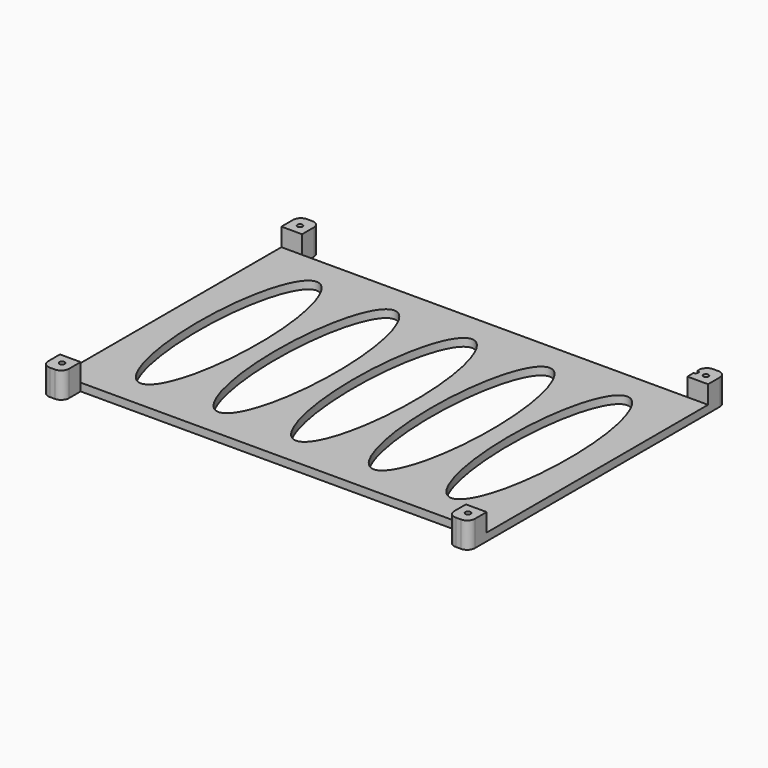
from build123d import *

# Parameters (mm, degrees)
F0_W     = 4
F0_H     = 106.96
F0_H_2   = 4
F0_W_2   = 148.9
F1_DEPTH = 3
F2_DEPTH = 10
F3_D     = 2
F5_DEPTH = 25


# Not quite as in the source:
# - a feature names something its author has since deleted; it is built from what else it names


with BuildPart() as f1:
    # F0 (on Top) → F1 (new body)
    with BuildSketch(Plane.XY):
        with Locations((-80.45, 0)):
            Rectangle(F0_W, F0_H)
        with Locations((-76.45, 55.48)):
            Rectangle(F0_W, F0_H_2)
        Rectangle(F0_W_2, F0_H)
        with Locations((-76.45, 0)):
            Rectangle(F0_W, F0_H)
        with BuildLine():
            ThreePointArc((82.45, 59.135), (81.5713203436, 61.2563203436), (79.45, 62.135))
            Line((79.45, 62.135), (77.45, 62.135))
            ThreePointArc((77.45, 62.135), (75.3286796564, 61.2563203436), (74.45, 59.135))
            Line((74.45, 59.135), (74.45, 57.48))
            Line((74.45, 57.48), (78.45, 57.48))
            Line((78.45, 57.48), (78.45, 53.48))
            Line((78.45, 53.48), (82.45, 53.48))
            Line((82.45, 53.48), (82.45, 59.135))
        make_face()
        with Locations((76.45, 55.48)):
            Rectangle(F0_W, F0_H_2)
        with Locations((76.45, 0)):
            Rectangle(F0_W, F0_H)
        with Locations((80.45, 0)):
            Rectangle(F0_W, F0_H)
        with Locations((76.45, -55.48)):
            Rectangle(F0_W, F0_H_2)
        with BuildLine():
            Line((82.45, -59.135), (82.45, -53.48))
            Line((82.45, -53.48), (78.45, -53.48))
            Line((78.45, -53.48), (78.45, -57.48))
            Line((78.45, -57.48), (74.45, -57.48))
            Line((74.45, -57.48), (74.45, -59.135))
            ThreePointArc((74.45, -59.135), (75.3286796564, -61.2563203436), (77.45, -62.135))
            Line((77.45, -62.135), (79.45, -62.135))
            ThreePointArc((79.45, -62.135), (81.5713203436, -61.2563203436), (82.45, -59.135))
        make_face()
        with BuildLine():
            Line((-78.45, -57.48), (-78.45, -53.48))
            Line((-78.45, -53.48), (-82.45, -53.48))
            Line((-82.45, -53.48), (-82.45, -59.135))
            ThreePointArc((-82.45, -59.135), (-81.5713203436, -61.2563203436), (-79.45, -62.135))
            Line((-79.45, -62.135), (-77.45, -62.135))
            ThreePointArc((-77.45, -62.135), (-75.3286796564, -61.2563203436), (-74.45, -59.135))
            Line((-74.45, -59.135), (-74.45, -57.48))
            Line((-74.45, -57.48), (-78.45, -57.48))
        make_face()
        with Locations((-76.45, -55.48)):
            Rectangle(F0_W, F0_H_2)
        with BuildLine():
            Line((-82.45, 53.48), (-78.45, 53.48))
            Line((-78.45, 53.48), (-78.45, 57.48))
            Line((-78.45, 57.48), (-74.45, 57.48))
            Line((-74.45, 57.48), (-74.45, 59.135))
            ThreePointArc((-74.45, 59.135), (-75.3286796564, 61.2563203436), (-77.45, 62.135))
            Line((-77.45, 62.135), (-79.45, 62.135))
            ThreePointArc((-79.45, 62.135), (-81.5713203436, 61.2563203436), (-82.45, 59.135))
            Line((-82.45, 59.135), (-82.45, 53.48))
        make_face()
    extrude(amount=F1_DEPTH)

    # F0 (on Top) → F2 (join)
    with BuildSketch(Plane.XY):
        with BuildLine():
            ThreePointArc((82.45, 59.135), (81.5713203436, 61.2563203436), (79.45, 62.135))
            Line((79.45, 62.135), (77.45, 62.135))
            ThreePointArc((77.45, 62.135), (75.3286796564, 61.2563203436), (74.45, 59.135))
            Line((74.45, 59.135), (74.45, 57.48))
            Line((74.45, 57.48), (78.45, 57.48))
            Line((78.45, 57.48), (78.45, 53.48))
            Line((78.45, 53.48), (82.45, 53.48))
            Line((82.45, 53.48), (82.45, 59.135))
        make_face()
        with Locations((76.45, 55.48)):
            Rectangle(F0_W, F0_H_2)
        with BuildLine():
            Line((-82.45, 53.48), (-78.45, 53.48))
            Line((-78.45, 53.48), (-78.45, 57.48))
            Line((-78.45, 57.48), (-74.45, 57.48))
            Line((-74.45, 57.48), (-74.45, 59.135))
            ThreePointArc((-74.45, 59.135), (-75.3286796564, 61.2563203436), (-77.45, 62.135))
            Line((-77.45, 62.135), (-79.45, 62.135))
            ThreePointArc((-79.45, 62.135), (-81.5713203436, 61.2563203436), (-82.45, 59.135))
            Line((-82.45, 59.135), (-82.45, 53.48))
        make_face()
        with Locations((-76.45, 55.48)):
            Rectangle(F0_W, F0_H_2)
        with BuildLine():
            Line((82.45, -59.135), (82.45, -53.48))
            Line((82.45, -53.48), (78.45, -53.48))
            Line((78.45, -53.48), (78.45, -57.48))
            Line((78.45, -57.48), (74.45, -57.48))
            Line((74.45, -57.48), (74.45, -59.135))
            ThreePointArc((74.45, -59.135), (75.3286796564, -61.2563203436), (77.45, -62.135))
            Line((77.45, -62.135), (79.45, -62.135))
            ThreePointArc((79.45, -62.135), (81.5713203436, -61.2563203436), (82.45, -59.135))
        make_face()
        with Locations((76.45, -55.48)):
            Rectangle(F0_W, F0_H_2)
        with BuildLine():
            Line((-78.45, -57.48), (-78.45, -53.48))
            Line((-78.45, -53.48), (-82.45, -53.48))
            Line((-82.45, -53.48), (-82.45, -59.135))
            ThreePointArc((-82.45, -59.135), (-81.5713203436, -61.2563203436), (-79.45, -62.135))
            Line((-79.45, -62.135), (-77.45, -62.135))
            ThreePointArc((-77.45, -62.135), (-75.3286796564, -61.2563203436), (-74.45, -59.135))
            Line((-74.45, -59.135), (-74.45, -57.48))
            Line((-74.45, -57.48), (-78.45, -57.48))
        make_face()
        with Locations((-76.45, -55.48)):
            Rectangle(F0_W, F0_H_2)
    extrude(amount=F2_DEPTH)

    # F3 (through all)
    with Locations(Plane(origin=(0, 0, 0), x_dir=(1, 0, 0), z_dir=(0, 0, -1))):
        with Locations((74.45, -57.48), (78.45, -57.48), (78.45, 57.48), (-78.45, 57.48), (-78.45, -57.48)):
            Hole(F3_D / 2)

    # F4 (on face) → F5 (cut)
    with BuildSketch(Plane.XY.offset(3)):
        with BuildLine():
            add(Edge.make_bspline(
                [(-60, 42.5), (-80.0186509611, 42.5), (-70.0093254806, -21.25), (-60, -85), (-49.9906745194, -21.25), (-39.9813490389, 42.5), (-60, 42.5)],
                knots=[0, 0, 0, 2.0943951024, 2.0943951024, 4.1887902048, 4.1887902048, 6.2831853072, 6.2831853072, 6.2831853072], degree=2, weights=[1, 0.5, 1, 0.5, 1, 0.5, 1]))
        make_face()
        with BuildLine():
            add(Edge.make_bspline(
                [(-30, 42.5), (-50.0186509611, 42.5), (-40.0093254806, -21.25), (-30, -85), (-19.9906745194, -21.25), (-9.9813490389, 42.5), (-30, 42.5)],
                knots=[0, 0, 0, 2.0943951024, 2.0943951024, 4.1887902048, 4.1887902048, 6.2831853072, 6.2831853072, 6.2831853072], degree=2, weights=[1, 0.5, 1, 0.5, 1, 0.5, 1]))
        make_face()
        with BuildLine():
            add(Edge.make_bspline(
                [(0, 42.5), (-20.0186509611, 42.5), (-10.0093254806, -21.25), (0, -85), (10.0093254806, -21.25), (20.0186509611, 42.5), (0, 42.5)],
                knots=[0, 0, 0, 2.0943951024, 2.0943951024, 4.1887902048, 4.1887902048, 6.2831853072, 6.2831853072, 6.2831853072], degree=2, weights=[1, 0.5, 1, 0.5, 1, 0.5, 1]))
        make_face()
        with BuildLine():
            add(Edge.make_bspline(
                [(30, 42.5), (9.9813490389, 42.5), (19.9906745194, -21.25), (30, -85), (40.0093254806, -21.25), (50.0186509611, 42.5), (30, 42.5)],
                knots=[0, 0, 0, 2.0943951024, 2.0943951024, 4.1887902048, 4.1887902048, 6.2831853072, 6.2831853072, 6.2831853072], degree=2, weights=[1, 0.5, 1, 0.5, 1, 0.5, 1]))
        make_face()
        with BuildLine():
            add(Edge.make_bspline(
                [(60, 42.5), (39.9813490389, 42.5), (49.9906745194, -21.25), (60, -85), (70.0093254806, -21.25), (80.0186509611, 42.5), (60, 42.5)],
                knots=[0, 0, 0, 2.0943951024, 2.0943951024, 4.1887902048, 4.1887902048, 6.2831853072, 6.2831853072, 6.2831853072], degree=2, weights=[1, 0.5, 1, 0.5, 1, 0.5, 1]))
        make_face()
    extrude(amount=-F5_DEPTH, mode=Mode.SUBTRACT)


solid = f1.part
